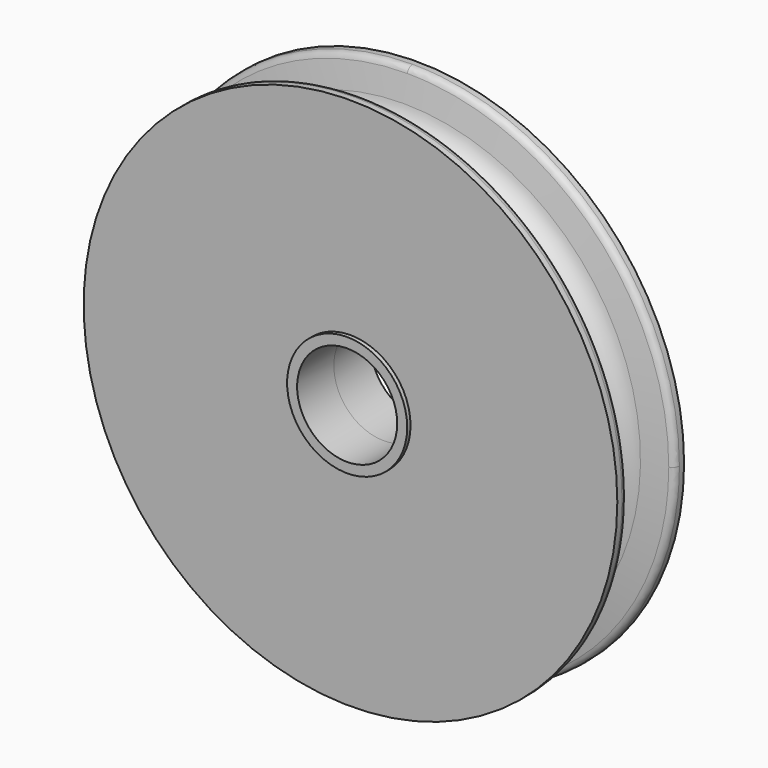
from build123d import *

# Parameters (mm, degrees)
F0_R          = 11.43
F0_R_2        = 9.525
F1_DEPTH      = 8.73125
F1_DEPTH_BACK = 8.7376
F0_R_3        = 50.8
F2_DEPTH      = 7.9375
F2_DEPTH_BACK = 7.9502
F5_R          = 1.27


with BuildPart() as f1:
    # F0 (on Front) → F1 (new body, two sides)
    with BuildSketch(Plane.XZ) as f1_sk:
        Circle(F0_R)
        Circle(F0_R_2, mode=Mode.SUBTRACT)
    extrude(amount=F1_DEPTH)
    extrude(f1_sk.sketch, amount=-F1_DEPTH_BACK)

    # F0 (on Front) → F2 (join, two sides)
    with BuildSketch(Plane.XZ) as f2_sk:
        Circle(F0_R_3)
        Circle(F0_R, mode=Mode.SUBTRACT)
    extrude(amount=F2_DEPTH)
    extrude(f2_sk.sketch, amount=-F2_DEPTH_BACK)

    # F3 (on Right) → F4 (revolve, cut)
    with BuildSketch(Plane.YZ):
        with BuildLine():
            Line((-6.35, 53.6575), (-4.6732280163, 45.1197058197))
            ThreePointArc((-4.6732280163, 45.1197058197), (0, 41.275), (4.6732280163, 45.1197058197))
            Line((4.6732280163, 45.1197058197), (6.35, 53.6575))
            Line((6.35, 53.6575), (0, 53.6575))
            Line((0, 53.6575), (-6.35, 53.6575))
        make_face()
    revolve(axis=Axis((0, 33.8884852827, 0), (0, 1, 0)), mode=Mode.SUBTRACT)

    # F5
    f5_edges = [f1.edges().sort_by_distance(p)[0] for p in [
        (35.921024, 5.788804, 35.921024),
        (-35.921024, 5.788804, -35.921024),
        (-35.921024, -5.788804, -35.921024),
        (35.921024, -5.788804, 35.921024),
    ]]
    fillet(f5_edges, radius=F5_R)


solid = f1.part
